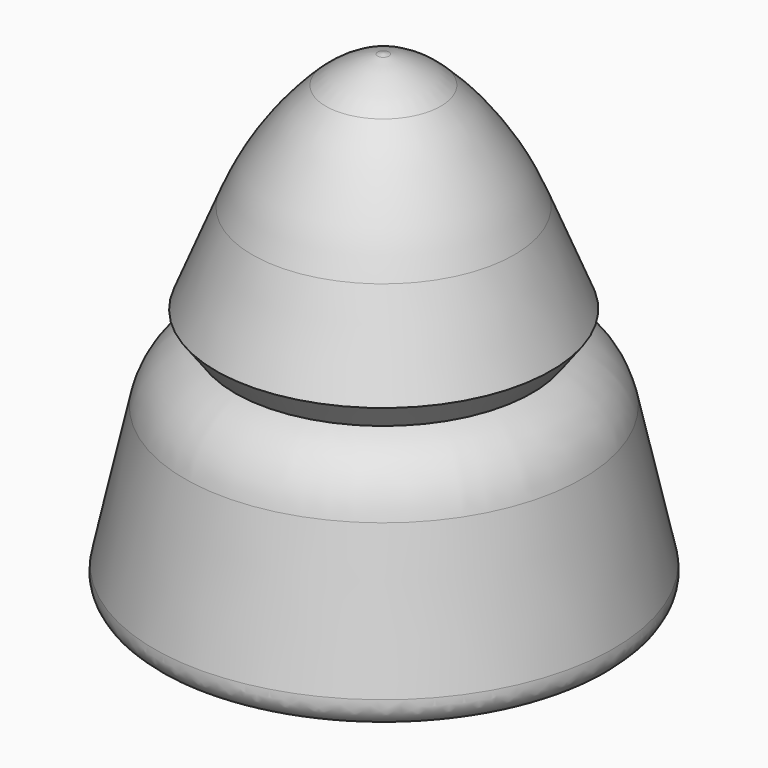
from build123d import *

# Parameters (mm, degrees)
F2_R = 10.8349837227
F3_R = 4.004166267
F4_R = 0.840522708


# Not quite as in the source:
# - a fillet or chamfer that OpenCascade refuses, or shapes differently, is made with other operations: its cross-section is extruded or revolved along the edge and cut away or added


with BuildPart() as f1:
    # F0 (on Front) → F1 (revolve)
    with BuildSketch(Plane.XZ):
        Polygon((-8.4658376873, 0), (0, 0), (-0.0272442667, 17.1914175153), (-1.2093468104, 16.9241316617), (-3.7246965803, 14.7794829682), (-6.0306731611, 9.0818414465), (-5.3430483676, 8.1584332511), (-6.7771640606, 7.7190031298), align=None)
    revolve(axis=Axis((-0.0136221333, 0, 8.5957087576), (0.0015847578, 0, -0.9999987443)))

    # F2
    f2_edges = [f1.edges().sort_by_distance(p)[0] for p in [
        (3.677834, 0, 14.791214),
    ]]
    fillet(f2_edges, radius=F2_R)

    # F3
    f3_edges = [f1.edges().sort_by_distance(p)[0] for p in [
        (1.1557, 0, 16.92788),
    ]]
    fillet(f3_edges, radius=F3_R)

    # F4
    f4_edges = [f1.edges().sort_by_distance(p)[0] for p in [
        (8.465795, 0, 0.026833),
    ]]
    fillet(f4_edges, radius=F4_R)

    # F5: fillet of radius 2.9679064036 on 1 edges, made by hand

    # F5_s1 → F5_t2 (revolve, cut)
    with BuildSketch(Plane.XZ):
        with BuildLine():
            ThreePointArc((-7.1455909431, 6.0349072725), (-6.5089088862, 7.3212652789), (-5.3430483676, 8.1584332511))
            Line((-5.3430483676, 8.1584332511), (-6.7771640606, 7.7190031298))
            Line((-6.7771640606, 7.7190031298), (-7.1455909431, 6.0349072725))
        make_face()
    revolve(axis=Axis((-0.0122497554, 0, 7.7297238937), (0.0015847578, 0, -0.9999987443)), mode=Mode.SUBTRACT)


solid = f1.part
